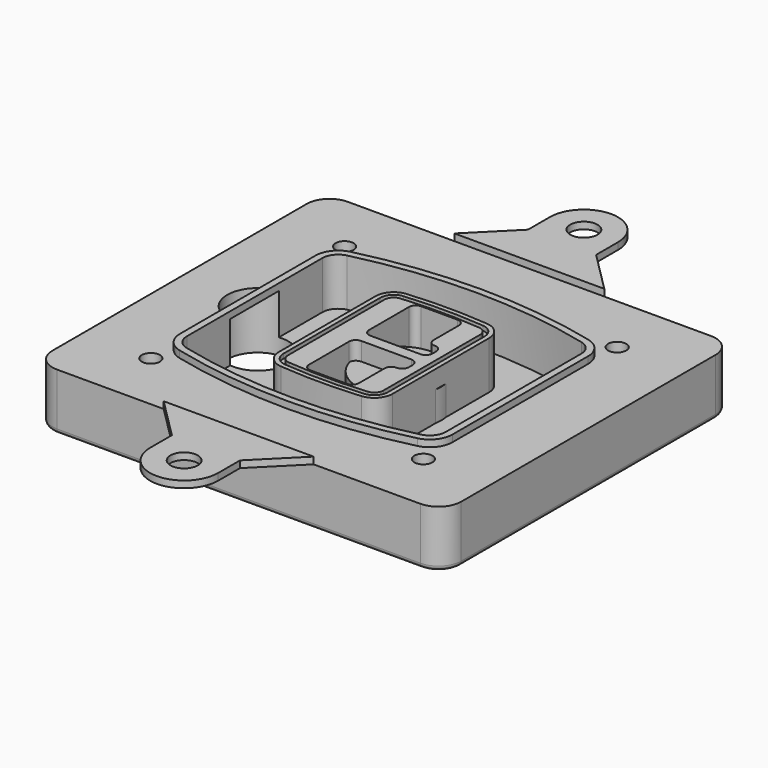
from build123d import *

# Parameters (mm, degrees)
F0_R      = 4
F1_DEPTH  = 25
F2_DEPTH  = 3
F3_DEPTH  = 18
F5_DEPTH  = 21
F6_DEPTH  = 2
F8_DEPTH  = 20
F9_DEPTH  = 16
F10_DEPTH = 25
F7_R      = 6
F7_R_2    = 4
F11_DEPTH = 6
F13_DEPTH = 9
F15_R     = 2
F16_R     = 6
F17_DEPTH = 3


# Not quite as in the source:
# - a feature of the source that left no trace in its solid (it failed there, or was rolled back) is left out
# - a feature names something its author has since deleted; it is built from what else it names


with BuildPart() as f1:
    # F0 (on Top) → F1 (new body)
    with BuildSketch(Plane.XY):
        with BuildLine():
            ThreePointArc((-90, -70), (-87.0710678119, -77.0710678119), (-80, -80))
            Line((-80, -80), (80, -80))
            ThreePointArc((80, -80), (87.0710678119, -77.0710678119), (90, -70))
            Line((90, -70), (90, 70))
            ThreePointArc((90, 70), (87.0710678119, 77.0710678119), (80, 80))
            Line((80, 80), (-80, 80))
            ThreePointArc((-80, 80), (-87.0710678119, 77.0710678119), (-90, 70))
            Line((-90, 70), (-90, -70))
        make_face()
        with Locations((-60, -53.3333333333)):
            Circle(F0_R, mode=Mode.SUBTRACT)
        with Locations((60, -53.3333333333)):
            Circle(F0_R, mode=Mode.SUBTRACT)
        with Locations((-60, 53.3333333333)):
            Circle(F0_R, mode=Mode.SUBTRACT)
        with BuildLine():
            ThreePointArc((-64, 37.2990447398), (-61.0143011354, 45.9411029726), (-53.3306899286, 50.8970778549))
            ThreePointArc((-53.3306899286, 50.8970778549), (0, 57.3333333333), (53.3306899286, 50.8970778549))
            ThreePointArc((53.3306899286, 50.8970778549), (61.0143011354, 45.9411029726), (64, 37.2990447398))
            Line((64, 37.2990447398), (64, -37.2990447398))
            ThreePointArc((64, -37.2990447398), (61.0143011354, -45.9411029726), (53.3306899286, -50.8970778549))
            ThreePointArc((53.3306899286, -50.8970778549), (0, -57.3333333333), (-53.3306899286, -50.8970778549))
            ThreePointArc((-53.3306899286, -50.8970778549), (-61.0143011354, -45.9411029726), (-64, -37.2990447398))
            Line((-64, -37.2990447398), (-64, 37.2990447398))
        make_face(mode=Mode.SUBTRACT)
        with Locations((60, 53.3333333333)):
            Circle(F0_R, mode=Mode.SUBTRACT)
        with BuildLine():
            ThreePointArc((53.3306899286, 50.8970778549), (0, 57.3333333333), (-53.3306899286, 50.8970778549))
            ThreePointArc((-53.3306899286, 50.8970778549), (-61.0143011354, 45.9411029726), (-64, 37.2990447398))
            Line((-64, 37.2990447398), (-64, -37.2990447398))
            ThreePointArc((-64, -37.2990447398), (-61.0143011354, -45.9411029726), (-53.3306899286, -50.8970778549))
            ThreePointArc((-53.3306899286, -50.8970778549), (0, -57.3333333333), (53.3306899286, -50.8970778549))
            ThreePointArc((53.3306899286, -50.8970778549), (61.0143011354, -45.9411029726), (64, -37.2990447398))
            Line((64, -37.2990447398), (64, 37.2990447398))
            ThreePointArc((64, 37.2990447398), (61.0143011354, 45.9411029726), (53.3306899286, 50.8970778549))
        make_face()
        with BuildLine():
            Line((-60, -37.2990447398), (-60, 37.2990447398))
            ThreePointArc((-60, 37.2990447398), (-57.8673579538, 43.4719434775), (-52.3790642347, 47.0119255363))
            ThreePointArc((-52.3790642347, 47.0119255363), (0, 53.3333333333), (52.3790642347, 47.0119255363))
            ThreePointArc((52.3790642347, 47.0119255363), (57.8673579538, 43.4719434775), (60, 37.2990447398))
            Line((60, 37.2990447398), (60, -37.2990447398))
            ThreePointArc((60, -37.2990447398), (57.8673579538, -43.4719434775), (52.3790642347, -47.0119255363))
            ThreePointArc((52.3790642347, -47.0119255363), (0, -53.3333333333), (-52.3790642347, -47.0119255363))
            ThreePointArc((-52.3790642347, -47.0119255363), (-57.8673579538, -43.4719434775), (-60, -37.2990447398))
        make_face(mode=Mode.SUBTRACT)
        with BuildLine():
            ThreePointArc((-52.3790642347, 47.0119255363), (-57.8673579538, 43.4719434775), (-60, 37.2990447398))
            Line((-60, 37.2990447398), (-60, -37.2990447398))
            ThreePointArc((-60, -37.2990447398), (-57.8673579538, -43.4719434775), (-52.3790642347, -47.0119255363))
            ThreePointArc((-52.3790642347, -47.0119255363), (0, -53.3333333333), (52.3790642347, -47.0119255363))
            ThreePointArc((52.3790642347, -47.0119255363), (57.8673579538, -43.4719434775), (60, -37.2990447398))
            Line((60, -37.2990447398), (60, 37.2990447398))
            ThreePointArc((60, 37.2990447398), (57.8673579538, 43.4719434775), (52.3790642347, 47.0119255363))
            ThreePointArc((52.3790642347, 47.0119255363), (0, 53.3333333333), (-52.3790642347, 47.0119255363))
        make_face()
        with BuildLine():
            ThreePointArc((51.6653449643, 44.0980612973), (55.5071505677, 41.6200738562), (57, 37.2990447398))
            Line((57, 37.2990447398), (57, -37.2990447398))
            ThreePointArc((57, -37.2990447398), (55.5071505677, -41.6200738562), (51.6653449643, -44.0980612973))
            ThreePointArc((51.6653449643, -44.0980612973), (0, -50.3333333333), (-51.6653449643, -44.0980612973))
            ThreePointArc((-51.6653449643, -44.0980612973), (-55.5071505677, -41.6200738562), (-57, -37.2990447398))
            Line((-57, -37.2990447398), (-57, 37.2990447398))
            ThreePointArc((-57, 37.2990447398), (-55.5071505677, 41.6200738562), (-51.6653449643, 44.0980612973))
            ThreePointArc((-51.6653449643, 44.0980612973), (0, 50.3333333333), (51.6653449643, 44.0980612973))
        make_face(mode=Mode.SUBTRACT)
        with BuildLine():
            Line((57, -37.2990447398), (57, 37.2990447398))
            ThreePointArc((57, 37.2990447398), (55.5071505677, 41.6200738562), (51.6653449643, 44.0980612973))
            ThreePointArc((51.6653449643, 44.0980612973), (0, 50.3333333333), (-51.6653449643, 44.0980612973))
            ThreePointArc((-51.6653449643, 44.0980612973), (-55.5071505677, 41.6200738562), (-57, 37.2990447398))
            Line((-57, 37.2990447398), (-57, -37.2990447398))
            ThreePointArc((-57, -37.2990447398), (-55.5071505677, -41.6200738562), (-51.6653449643, -44.0980612973))
            ThreePointArc((-51.6653449643, -44.0980612973), (0, -50.3333333333), (51.6653449643, -44.0980612973))
            ThreePointArc((51.6653449643, -44.0980612973), (55.5071505677, -41.6200738562), (57, -37.2990447398))
        make_face()
    extrude(amount=-F1_DEPTH)

    # F0 (on Top) → F2 (join)
    with BuildSketch(Plane.XY):
        with BuildLine():
            ThreePointArc((-52.3790642347, 47.0119255363), (-57.8673579538, 43.4719434775), (-60, 37.2990447398))
            Line((-60, 37.2990447398), (-60, -37.2990447398))
            ThreePointArc((-60, -37.2990447398), (-57.8673579538, -43.4719434775), (-52.3790642347, -47.0119255363))
            ThreePointArc((-52.3790642347, -47.0119255363), (0, -53.3333333333), (52.3790642347, -47.0119255363))
            ThreePointArc((52.3790642347, -47.0119255363), (57.8673579538, -43.4719434775), (60, -37.2990447398))
            Line((60, -37.2990447398), (60, 37.2990447398))
            ThreePointArc((60, 37.2990447398), (57.8673579538, 43.4719434775), (52.3790642347, 47.0119255363))
            ThreePointArc((52.3790642347, 47.0119255363), (0, 53.3333333333), (-52.3790642347, 47.0119255363))
        make_face()
        with BuildLine():
            ThreePointArc((51.6653449643, 44.0980612973), (55.5071505677, 41.6200738562), (57, 37.2990447398))
            Line((57, 37.2990447398), (57, -37.2990447398))
            ThreePointArc((57, -37.2990447398), (55.5071505677, -41.6200738562), (51.6653449643, -44.0980612973))
            ThreePointArc((51.6653449643, -44.0980612973), (0, -50.3333333333), (-51.6653449643, -44.0980612973))
            ThreePointArc((-51.6653449643, -44.0980612973), (-55.5071505677, -41.6200738562), (-57, -37.2990447398))
            Line((-57, -37.2990447398), (-57, 37.2990447398))
            ThreePointArc((-57, 37.2990447398), (-55.5071505677, 41.6200738562), (-51.6653449643, 44.0980612973))
            ThreePointArc((-51.6653449643, 44.0980612973), (0, 50.3333333333), (51.6653449643, 44.0980612973))
        make_face(mode=Mode.SUBTRACT)
    extrude(amount=F2_DEPTH)

    # F0 (on Top) → F3 (cut)
    with BuildSketch(Plane.XY):
        with BuildLine():
            Line((57, -37.2990447398), (57, 37.2990447398))
            ThreePointArc((57, 37.2990447398), (55.5071505677, 41.6200738562), (51.6653449643, 44.0980612973))
            ThreePointArc((51.6653449643, 44.0980612973), (0, 50.3333333333), (-51.6653449643, 44.0980612973))
            ThreePointArc((-51.6653449643, 44.0980612973), (-55.5071505677, 41.6200738562), (-57, 37.2990447398))
            Line((-57, 37.2990447398), (-57, -37.2990447398))
            ThreePointArc((-57, -37.2990447398), (-55.5071505677, -41.6200738562), (-51.6653449643, -44.0980612973))
            ThreePointArc((-51.6653449643, -44.0980612973), (0, -50.3333333333), (51.6653449643, -44.0980612973))
            ThreePointArc((51.6653449643, -44.0980612973), (55.5071505677, -41.6200738562), (57, -37.2990447398))
        make_face()
    extrude(amount=-F3_DEPTH, mode=Mode.SUBTRACT)

    # F4 (on face) → F5 (join, through all)
    with BuildSketch(Plane.XY.offset(3)):
        with BuildLine():
            ThreePointArc((-25, -26.587695628), (-22.8992979869, -31.9912392117), (-17.7004291845, -34.5569740744))
            ThreePointArc((-17.7004291845, -34.5569740744), (0, -35.3333333333), (17.7004291845, -34.5569740744))
            ThreePointArc((17.7004291845, -34.5569740744), (22.8992979869, -31.9912392117), (25, -26.587695628))
            Line((25, -26.587695628), (25, 26.587695628))
            ThreePointArc((25, 26.587695628), (22.8992979869, 31.9912392117), (17.7004291845, 34.5569740744))
            ThreePointArc((17.7004291845, 34.5569740744), (0, 35.3333333333), (-17.7004291845, 34.5569740744))
            ThreePointArc((-17.7004291845, 34.5569740744), (-22.8992979869, 31.9912392117), (-25, 26.587695628))
            Line((-25, 26.587695628), (-25, -26.587695628))
        make_face()
        with BuildLine():
            ThreePointArc((17.5253218884, 32.5646544628), (21.4244734902, 30.6403533158), (23, 26.587695628))
            Line((23, 26.587695628), (23, -26.587695628))
            ThreePointArc((23, -26.587695628), (21.4244734902, -30.6403533158), (17.5253218884, -32.5646544628))
            ThreePointArc((17.5253218884, -32.5646544628), (0, -33.3333333333), (-17.5253218884, -32.5646544628))
            ThreePointArc((-17.5253218884, -32.5646544628), (-21.4244734902, -30.6403533158), (-23, -26.587695628))
            Line((-23, -26.587695628), (-23, 26.587695628))
            ThreePointArc((-23, 26.587695628), (-21.4244734902, 30.6403533158), (-17.5253218884, 32.5646544628))
            ThreePointArc((-17.5253218884, 32.5646544628), (0, 33.3333333333), (17.5253218884, 32.5646544628))
        make_face(mode=Mode.SUBTRACT)
        with BuildLine():
            Line((23, -26.587695628), (23, 26.587695628))
            ThreePointArc((23, 26.587695628), (21.4244734902, 30.6403533158), (17.5253218884, 32.5646544628))
            ThreePointArc((17.5253218884, 32.5646544628), (0, 33.3333333333), (-17.5253218884, 32.5646544628))
            ThreePointArc((-17.5253218884, 32.5646544628), (-21.4244734902, 30.6403533158), (-23, 26.587695628))
            Line((-23, 26.587695628), (-23, -26.587695628))
            ThreePointArc((-23, -26.587695628), (-21.4244734902, -30.6403533158), (-17.5253218884, -32.5646544628))
            ThreePointArc((-17.5253218884, -32.5646544628), (0, -33.3333333333), (17.5253218884, -32.5646544628))
            ThreePointArc((17.5253218884, -32.5646544628), (21.4244734902, -30.6403533158), (23, -26.587695628))
        make_face()
        with BuildLine():
            ThreePointArc((17.3502145923, 30.5723348512), (19.9496489934, 29.2894674198), (21, 26.587695628))
            Line((21, 26.587695628), (21, -26.587695628))
            ThreePointArc((21, -26.587695628), (19.9496489934, -29.2894674198), (17.3502145923, -30.5723348512))
            ThreePointArc((17.3502145923, -30.5723348512), (0, -31.3333333333), (-17.3502145923, -30.5723348512))
            ThreePointArc((-17.3502145923, -30.5723348512), (-19.9496489934, -29.2894674198), (-21, -26.587695628))
            Line((-21, -26.587695628), (-21, 26.587695628))
            ThreePointArc((-21, 26.587695628), (-19.9496489934, 29.2894674198), (-17.3502145923, 30.5723348512))
            ThreePointArc((-17.3502145923, 30.5723348512), (0, 31.3333333333), (17.3502145923, 30.5723348512))
        make_face(mode=Mode.SUBTRACT)
        with BuildLine():
            Line((21, -26.587695628), (21, 26.587695628))
            ThreePointArc((21, 26.587695628), (19.9496489934, 29.2894674198), (17.3502145923, 30.5723348512))
            ThreePointArc((17.3502145923, 30.5723348512), (0, 31.3333333333), (-17.3502145923, 30.5723348512))
            ThreePointArc((-17.3502145923, 30.5723348512), (-19.9496489934, 29.2894674198), (-21, 26.587695628))
            Line((-21, 26.587695628), (-21, -26.587695628))
            ThreePointArc((-21, -26.587695628), (-19.9496489934, -29.2894674198), (-17.3502145923, -30.5723348512))
            ThreePointArc((-17.3502145923, -30.5723348512), (0, -31.3333333333), (17.3502145923, -30.5723348512))
            ThreePointArc((17.3502145923, -30.5723348512), (19.9496489934, -29.2894674198), (21, -26.587695628))
        make_face()
        with BuildLine():
            Line((-8, -2.5), (14, -2.5))
            ThreePointArc((14, -2.5), (16.1213203436, -3.3786796564), (17, -5.5))
            Line((17, -5.5), (17, -7.5))
            ThreePointArc((17, -7.5), (16.1213203436, -9.6213203436), (14, -10.5))
            ThreePointArc((14, -10.5), (11.8786796564, -11.3786796564), (11, -13.5))
            Line((11, -13.5), (11, -27.5))
            ThreePointArc((11, -27.5), (10.1213203436, -29.6213203436), (8, -30.5))
            Line((8, -30.5), (-8, -30.5))
            ThreePointArc((-8, -30.5), (-10.1213203436, -29.6213203436), (-11, -27.5))
            Line((-11, -27.5), (-11, -5.5))
            ThreePointArc((-11, -5.5), (-10.1213203436, -3.3786796564), (-8, -2.5))
        make_face(mode=Mode.SUBTRACT)
        with BuildLine():
            ThreePointArc((-8, 2.5), (-10.1213203436, 3.3786796564), (-11, 5.5))
            Line((-11, 5.5), (-11, 27.5))
            ThreePointArc((-11, 27.5), (-10.1213203436, 29.6213203436), (-8, 30.5))
            Line((-8, 30.5), (8, 30.5))
            ThreePointArc((8, 30.5), (10.1213203436, 29.6213203436), (11, 27.5))
            Line((11, 27.5), (11, 13.5))
            ThreePointArc((11, 13.5), (11.8786796564, 11.3786796564), (14, 10.5))
            ThreePointArc((14, 10.5), (16.1213203436, 9.6213203436), (17, 7.5))
            Line((17, 7.5), (17, 5.5))
            ThreePointArc((17, 5.5), (16.1213203436, 3.3786796564), (14, 2.5))
            Line((14, 2.5), (-8, 2.5))
        make_face(mode=Mode.SUBTRACT)
    extrude(amount=-F5_DEPTH)

    # F4 (on face) → F6 (cut)
    with BuildSketch(Plane.XY.offset(3)):
        with BuildLine():
            Line((23, -26.587695628), (23, 26.587695628))
            ThreePointArc((23, 26.587695628), (21.4244734902, 30.6403533158), (17.5253218884, 32.5646544628))
            ThreePointArc((17.5253218884, 32.5646544628), (0, 33.3333333333), (-17.5253218884, 32.5646544628))
            ThreePointArc((-17.5253218884, 32.5646544628), (-21.4244734902, 30.6403533158), (-23, 26.587695628))
            Line((-23, 26.587695628), (-23, -26.587695628))
            ThreePointArc((-23, -26.587695628), (-21.4244734902, -30.6403533158), (-17.5253218884, -32.5646544628))
            ThreePointArc((-17.5253218884, -32.5646544628), (0, -33.3333333333), (17.5253218884, -32.5646544628))
            ThreePointArc((17.5253218884, -32.5646544628), (21.4244734902, -30.6403533158), (23, -26.587695628))
        make_face()
        with BuildLine():
            ThreePointArc((17.3502145923, 30.5723348512), (19.9496489934, 29.2894674198), (21, 26.587695628))
            Line((21, 26.587695628), (21, -26.587695628))
            ThreePointArc((21, -26.587695628), (19.9496489934, -29.2894674198), (17.3502145923, -30.5723348512))
            ThreePointArc((17.3502145923, -30.5723348512), (0, -31.3333333333), (-17.3502145923, -30.5723348512))
            ThreePointArc((-17.3502145923, -30.5723348512), (-19.9496489934, -29.2894674198), (-21, -26.587695628))
            Line((-21, -26.587695628), (-21, 26.587695628))
            ThreePointArc((-21, 26.587695628), (-19.9496489934, 29.2894674198), (-17.3502145923, 30.5723348512))
            ThreePointArc((-17.3502145923, 30.5723348512), (0, 31.3333333333), (17.3502145923, 30.5723348512))
        make_face(mode=Mode.SUBTRACT)
    extrude(amount=-F6_DEPTH, mode=Mode.SUBTRACT)

    # F7 (on face) → F8 (join)
    with BuildSketch(Plane(origin=(0, 0, -25), x_dir=(1, 0, 0), z_dir=(0, 0, -1))):
        with BuildLine():
            ThreePointArc((-6.71157564, 0), (6.7567035675, 13.4682792075), (20.224982775, 0))
            Line((20.224982775, 0), (25.224982775, 0))
            ThreePointArc((25.224982775, 0), (6.7567035675, 18.4682792075), (-11.71157564, 0))
            Line((-11.71157564, 0), (-6.71157564, 0))
        make_face()
        with BuildLine():
            Line((-6.71157564, 0), (20.224982775, 0))
            ThreePointArc((20.224982775, 0), (6.7567035675, 13.4682792075), (-6.71157564, 0))
        make_face()
        with BuildLine():
            ThreePointArc((-6.71157564, 0), (6.7567035675, -13.4682792075), (20.224982775, 0))
            Line((20.224982775, 0), (-6.71157564, 0))
        make_face()
        with BuildLine():
            Line((25.224982775, 0), (20.224982775, 0))
            ThreePointArc((20.224982775, 0), (6.7567035675, -13.4682792075), (-6.71157564, 0))
            Line((-6.71157564, 0), (-11.71157564, 0))
            ThreePointArc((-11.71157564, 0), (6.7567035675, -18.4682792075), (25.224982775, 0))
        make_face()
    extrude(amount=-F8_DEPTH)

    # F7 (on face) → F9 (cut)
    with BuildSketch(Plane(origin=(0, 0, -25), x_dir=(1, 0, 0), z_dir=(0, 0, -1))):
        with BuildLine():
            Line((-6.71157564, 0), (20.224982775, 0))
            ThreePointArc((20.224982775, 0), (6.7567035675, 13.4682792075), (-6.71157564, 0))
        make_face()
        with BuildLine():
            ThreePointArc((-6.71157564, 0), (6.7567035675, -13.4682792075), (20.224982775, 0))
            Line((20.224982775, 0), (-6.71157564, 0))
        make_face()
    extrude(amount=-F9_DEPTH, mode=Mode.SUBTRACT)

    # F7 (on face) → F10 (cut)
    with BuildSketch(Plane(origin=(0, 0, -25), x_dir=(1, 0, 0), z_dir=(0, 0, -1))):
        with BuildLine():
            Line((-69.0318229325, 0), (-42.0952645175, 0))
            ThreePointArc((-42.0952645175, 0), (-55.563543725, 13.4682792075), (-69.0318229325, 0))
        make_face()
        with BuildLine():
            ThreePointArc((-69.0318229325, 0), (-55.563543725, -13.4682792075), (-42.0952645175, 0))
            Line((-42.0952645175, 0), (-69.0318229325, 0))
        make_face()
    extrude(amount=-F10_DEPTH, mode=Mode.SUBTRACT)

    # F7 (on face) → F11 (cut)
    with BuildSketch(Plane(origin=(0, 0, -25), x_dir=(1, 0, 0), z_dir=(0, 0, -1))):
        with Locations((60, -53.3333333333)):
            Circle(F7_R)
        with Locations((60, -53.3333333333)):
            Circle(F7_R_2, mode=Mode.SUBTRACT)
        with Locations((-60, -53.3333333333)):
            Circle(F7_R)
        with Locations((-60, -53.3333333333)):
            Circle(F7_R_2, mode=Mode.SUBTRACT)
        with Locations((-60, 53.3333333333)):
            Circle(F7_R)
        with Locations((-60, 53.3333333333)):
            Circle(F7_R_2, mode=Mode.SUBTRACT)
        with Locations((60, 53.3333333333)):
            Circle(F7_R)
        with Locations((60, 53.3333333333)):
            Circle(F7_R_2, mode=Mode.SUBTRACT)
    extrude(amount=-F11_DEPTH, mode=Mode.SUBTRACT)

    # F12 (on face) → F13 (cut, through all)
    with BuildSketch(Plane(origin=(0, 0, -9), x_dir=(1, 0, 0), z_dir=(0, 0, -1))):
        with BuildLine():
            ThreePointArc((20.224982775, 0), (20.1663399806, 1.2554664788), (19.9909222755, 2.5))
            Line((19.9909222755, 2.5), (14, 2.5))
            ThreePointArc((14, 2.5), (16.1213203436, 3.3786796564), (17, 5.5))
            Line((17, 5.5), (17, 7.5))
            ThreePointArc((17, 7.5), (16.1213203436, 9.6213203436), (14, 10.5))
            ThreePointArc((14, 10.5), (12.1627255951, 11.1284134507), (11.0951631559, 12.750384826))
            ThreePointArc((11.0951631559, 12.750384826), (11.0476113807, 12.7664660322), (11, 12.7823698976))
            Line((11, 12.7823698976), (11, -12.7823698976))
            ThreePointArc((11, -12.7823698976), (11.0476113807, -12.7664660322), (11.0951631559, -12.750384826))
            ThreePointArc((11.0951631559, -12.750384826), (12.1627255951, -11.1284134507), (14, -10.5))
            ThreePointArc((14, -10.5), (16.1213203436, -9.6213203436), (17, -7.5))
            Line((17, -7.5), (17, -5.5))
            ThreePointArc((17, -5.5), (16.1213203436, -3.3786796564), (14, -2.5))
            Line((14, -2.5), (19.9909222755, -2.5))
            ThreePointArc((19.9909222755, -2.5), (20.1663399806, -1.2554664788), (20.224982775, 0))
        make_face()
    extrude(amount=F13_DEPTH, mode=Mode.SUBTRACT)

    # F15
    f15_edges = [f1.edges().sort_by_distance(p)[0] for p in [
        (0, -80, -25),
        (-90, 0, -25),
        (-87.071068, 77.071068, -25),
        (-87.071068, -77.071068, -25),
        (0, 80, -25),
        (87.071068, 77.071068, -25),
        (87.071068, -77.071068, -25),
        (90, 0, -25),
    ]]
    fillet(f15_edges, radius=F15_R)


with BuildPart() as f17:
    # F16 (on face) → F17 (new body, through all)
    with BuildSketch(Plane.XY):
        with BuildLine():
            Line((15, 98), (15, 110))
            ThreePointArc((15, 110), (0, 125), (-15, 110))
            Line((-15, 110), (-15, 98))
            Line((-15, 98), (-33, 80))
            Line((-33, 80), (33, 80))
            Line((33, 80), (15, 98))
        make_face()
        with Locations((0, 110)):
            Circle(F16_R, mode=Mode.SUBTRACT)
    extrude(amount=F17_DEPTH)


with BuildPart() as f17b:
    # F16 (on face) → F17, piece 2 (new body, through all)
    with BuildSketch(Plane.XY):
        with BuildLine():
            Line((15, -98), (33, -80))
            Line((33, -80), (-33, -80))
            Line((-33, -80), (-15, -98))
            Line((-15, -98), (-15, -110))
            ThreePointArc((-15, -110), (0, -125), (15, -110))
            Line((15, -110), (15, -98))
        make_face()
        with Locations((0, -110)):
            Circle(F16_R, mode=Mode.SUBTRACT)
    extrude(amount=F17_DEPTH)


solid = Compound([f1.part, f17.part, f17b.part])
